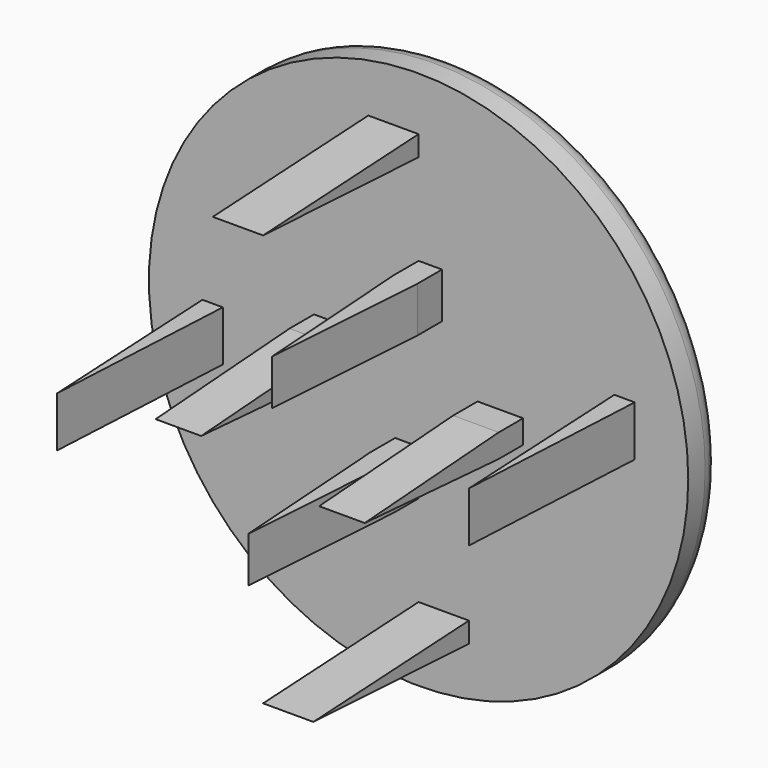
from build123d import *

# Parameters (mm, degrees)
F0_R         = 67.2715048221
F1_DEPTH     = 25.4
F2_SIZE2     = 47.9485215904
F2_SIZE      = 16.51
F3_DEPTH     = 7.62
F4_R         = 25.9737658724
F5_DEPTH     = 12.7
F6_W         = 12.5492112711
F6_H         = 5.0823129714
F6_W_2       = 5.8439155109
F6_H_2       = 11.3746980205
F6_W_3       = 5.0823129714
F6_H_3       = 12.5492112711
F6_W_4       = 11.3746980205
F6_H_4       = 5.8439155109
F7_DEPTH     = 50.8
F8_T4_DEPTH  = 276.6958225406
F8_T9_DEPTH  = 276.6958225406
F9_T4_DEPTH  = 235.8904693574
F9_T9_DEPTH  = 235.8904693574
F10_T1_DEPTH = 123.632583689
F11_T4_DEPTH = 235.8904693574
F11_T9_DEPTH = 235.8904693574
F12_T4_DEPTH = 235.8904693574
F12_T9_DEPTH = 235.8904693574
F13_T4_DEPTH = 276.6958225406
F13_T9_DEPTH = 276.6958225406
F14_T4_DEPTH = 276.6958225406
F14_T9_DEPTH = 276.6958225406
F15_T4_DEPTH = 276.6958225406
F15_T9_DEPTH = 276.6958225406
F16_R        = 5.08
F17_R        = 1.27


# Not quite as in the source:
# - a fillet or chamfer that OpenCascade refuses, or shapes differently, is made with other operations: its cross-section is extruded or revolved along the edge and cut away or added


with BuildPart() as f1:
    # F0 (on Front) → F1 (new body)
    with BuildSketch(Plane.XZ):
        Circle(F0_R)
    extrude(amount=-F1_DEPTH)

    # F2
    f2_edges = [f1.edges().sort_by_distance(p)[0] for p in [
        (-67.271505, 25.4, 0),
    ]]
    f2_side = f1.faces().sort_by_distance((-67.271505, 12.7, 0))[0]
    chamfer(f2_edges, length=F2_SIZE, length2=F2_SIZE2, reference=f2_side)

    # F3 (add): a face of the model
    f3_faces = [f1.faces().sort_by_distance(p)[0] for p in [
        (0, 25.4, 0),
    ]]
    extrude(f3_faces, amount=F3_DEPTH)

    # F4 (on face) → F5 (join)
    with BuildSketch(Plane(origin=(0, 33.02, 0), x_dir=(-1, 0, 0), z_dir=(0, 1, 0))):
        Circle(F4_R)
    extrude(amount=F5_DEPTH)

    # F6 (on face) → F7 (join)
    with BuildSketch(Plane.XZ):
        with Locations((-6.2746056356, 51.3789299875)):
            Rectangle(F6_W, F6_H)
        with Locations((2.9219577555, 20.4010321759)):
            Rectangle(F6_W_2, F6_H_2)
        with Locations((-51.3789299875, -6.2746056356)):
            Rectangle(F6_W_3, F6_H_3)
        with Locations((-20.4010321759, 2.9219577555)):
            Rectangle(F6_W_4, F6_H_4)
        with Locations((6.2746056356, -51.3789299875)):
            Rectangle(F6_W, F6_H)
        with Locations((-2.9219577555, -20.4010321759)):
            Rectangle(F6_W_2, F6_H_2)
        with Locations((51.3789299875, 6.2746056356)):
            Rectangle(F6_W_3, F6_H_3)
        with Locations((20.4010321759, -2.9219577555)):
            Rectangle(F6_W_4, F6_H_4)
    extrude(amount=F7_DEPTH)

    # F8: chamfer of 50.8 x 2.6623151876 on 2 edges, made by hand


with BuildPart() as f8_tool2:
    # F8_s3 → F8_t4 (new body)
    with BuildSketch(Plane.YZ.offset(132.0733056347)):
        Polygon((0, 53.9200864732), (-50.8, 51.2577712856), (-50.8, 53.9200864732), align=None)
    extrude(amount=-F8_T4_DEPTH)

    split(bisect_by=Plane.XZ, keep=Keep.TOP)


with BuildPart() as f1_1:
    add(f1.part)

    # F8_t1: cut F8_tool2
    add(f8_tool2.part, mode=Mode.SUBTRACT)


with BuildPart() as f8_tool7:
    # F8_s8 → F8_t9 (new body)
    with BuildSketch(Plane.YZ.offset(-144.6225169058)):
        Polygon((0, 48.8377735019), (-50.8, 51.5000886895), (-50.8, 48.8377735019), align=None)
    extrude(amount=F8_T9_DEPTH)

    split(bisect_by=Plane.XZ, keep=Keep.TOP)


with BuildPart() as f1_2:
    add(f1_1.part)

    # F8_t6: cut F8_tool7
    add(f8_tool7.part, mode=Mode.SUBTRACT)

    # F9: chamfer of 43.18 x 3.0194397397 on 2 edges, made by hand


with BuildPart() as f9_tool2:
    # F9_s3 → F9_t4 (new body)
    with BuildSketch(Plane.XY.offset(-97.5442025028)):
        Polygon((2.8244757712, -50.8), (5.8439155109, -7.62), (5.8439155109, -50.8), align=None)
    extrude(amount=F9_T4_DEPTH)

    split(bisect_by=Plane.XY.offset(-48.8377735019), keep=Keep.TOP)


with BuildPart() as f1_3:
    add(f1_2.part)

    # F9_t1: cut F9_tool2
    add(f9_tool2.part, mode=Mode.SUBTRACT)


with BuildPart() as f9_tool7:
    # F9_s8 → F9_t9 (new body)
    with BuildSketch(Plane.XY.offset(138.3462668546)):
        Polygon((3.0194397397, -50.8), (0, -7.62), (0, -50.8), align=None)
    extrude(amount=-F9_T9_DEPTH)

    split(bisect_by=Plane.XY.offset(-26.0883811861), keep=Keep.TOP)


with BuildPart() as f1_4:
    add(f1_3.part)

    # F9_t6: cut F9_tool7
    add(f9_tool7.part, mode=Mode.SUBTRACT)

    # F10: chamfer of 43.18 x 3.0194397397 on 2 edges, made by hand

    # F10_s2 → F10_t1 (cut)
    with BuildSketch(Plane.YZ.offset(-138.3462668546)):
        Polygon((-7.62, 0), (-50.8, 3.0194397397), (-50.8, 0), align=None)
        Polygon((-50.8, 2.8244757712), (-7.62, 5.8439155109), (-50.8, 5.8439155109), align=None)
    extrude(amount=F10_T1_DEPTH, mode=Mode.SUBTRACT)

    # F11: chamfer of 43.18 x 3.0194397397 on 2 edges, made by hand


with BuildPart() as f11_tool2:
    # F11_s3 → F11_t4 (new body)
    with BuildSketch(Plane.XY.offset(97.5442025028)):
        Polygon((-2.8244757712, -50.8), (-5.8439155109, -7.62), (-5.8439155109, -50.8), align=None)
    extrude(amount=-F11_T4_DEPTH)

    split(bisect_by=Plane(origin=(0, 2.5524687068, 48.7040042853), x_dir=(1, 0, 0), z_dir=(0, -0.0523359562, -0.9986295348)), keep=Keep.TOP)


with BuildPart() as f1_5:
    add(f1_4.part)

    # F11_t1: cut F11_tool2
    add(f11_tool2.part, mode=Mode.SUBTRACT)


with BuildPart() as f11_tool7:
    # F11_s8 → F11_t9 (new body)
    with BuildSketch(Plane.XY.offset(-138.3462668546)):
        Polygon((0, -7.62), (-3.0194397397, -50.8), (0, -50.8), align=None)
    extrude(amount=F11_T9_DEPTH)

    split(bisect_by=Plane(origin=(0, 2.5524687068, 48.7040042853), x_dir=(1, 0, 0), z_dir=(0, -0.0523359562, -0.9986295348)), keep=Keep.TOP)


with BuildPart() as f1_6:
    add(f1_5.part)

    # F11_t6: cut F11_tool7
    add(f11_tool7.part, mode=Mode.SUBTRACT)

    # F12: chamfer of 43.18 x 3.0194397397 on 2 edges, made by hand


with BuildPart() as f12_tool2:
    # F12_s3 → F12_t4 (new body)
    with BuildSketch(Plane.YZ.offset(-97.5442025028)):
        Polygon((-50.8, -2.8244757712), (-7.62, -5.8439155109), (-50.8, -5.8439155109), align=None)
    extrude(amount=F12_T4_DEPTH)

    split(bisect_by=Plane.YZ.offset(-48.8377735019), keep=Keep.TOP)


with BuildPart() as f1_7:
    add(f1_6.part)

    # F12_t1: cut F12_tool2
    add(f12_tool2.part, mode=Mode.SUBTRACT)


with BuildPart() as f12_tool7:
    # F12_s8 → F12_t9 (new body)
    with BuildSketch(Plane.YZ.offset(138.3462668546)):
        Polygon((-7.62, 0), (-50.8, -3.0194397397), (-50.8, 0), align=None)
    extrude(amount=-F12_T9_DEPTH)

    split(bisect_by=Plane.YZ.offset(-48.8377735019), keep=Keep.TOP)


with BuildPart() as f1_8:
    add(f1_7.part)

    # F12_t6: cut F12_tool7
    add(f12_tool7.part, mode=Mode.SUBTRACT)

    # F13: chamfer of 50.8 x 2.6623151876 on 2 edges, made by hand


with BuildPart() as f13_tool2:
    # F13_s3 → F13_t4 (new body)
    with BuildSketch(Plane.XY.offset(132.0733056347)):
        Polygon((-51.5000886895, -50.8), (-48.8377735019, 0), (-48.8377735019, -50.8), align=None)
    extrude(amount=-F13_T4_DEPTH)

    split(bisect_by=Plane.XZ, keep=Keep.TOP)


with BuildPart() as f1_9:
    add(f1_8.part)

    # F13_t1: cut F13_tool2
    add(f13_tool2.part, mode=Mode.SUBTRACT)


with BuildPart() as f13_tool7:
    # F13_s8 → F13_t9 (new body)
    with BuildSketch(Plane.XY.offset(132.0733056347)):
        Polygon((-51.2577712856, -50.8), (-53.9200864732, 0), (-53.9200864732, -50.8), align=None)
    extrude(amount=-F13_T9_DEPTH)

    split(bisect_by=Plane.XZ, keep=Keep.TOP)


with BuildPart() as f1_10:
    add(f1_9.part)

    # F13_t6: cut F13_tool7
    add(f13_tool7.part, mode=Mode.SUBTRACT)

    # F14: chamfer of 50.8 x 2.6623151876 on 2 edges, made by hand


with BuildPart() as f14_tool2:
    # F14_s3 → F14_t4 (new body)
    with BuildSketch(Plane.YZ.offset(-132.0733056347)):
        Polygon((-50.8, -51.2577712856), (0, -53.9200864732), (-50.8, -53.9200864732), align=None)
    extrude(amount=F14_T4_DEPTH)

    split(bisect_by=Plane.XZ, keep=Keep.TOP)


with BuildPart() as f1_11:
    add(f1_10.part)

    # F14_t1: cut F14_tool2
    add(f14_tool2.part, mode=Mode.SUBTRACT)


with BuildPart() as f14_tool7:
    # F14_s8 → F14_t9 (new body)
    with BuildSketch(Plane.YZ.offset(-132.0733056347)):
        Polygon((-50.8, -51.5000886895), (0, -48.8377735019), (-50.8, -48.8377735019), align=None)
    extrude(amount=F14_T9_DEPTH)

    split(bisect_by=Plane.XZ, keep=Keep.TOP)


with BuildPart() as f1_12:
    add(f1_11.part)

    # F14_t6: cut F14_tool7
    add(f14_tool7.part, mode=Mode.SUBTRACT)

    # F15: chamfer of 50.8 x 2.6623151876 on 2 edges, made by hand


with BuildPart() as f15_tool2:
    # F15_s3 → F15_t4 (new body)
    with BuildSketch(Plane.XY.offset(-132.0733056347)):
        Polygon((51.2577712856, -50.8), (53.9200864732, 0), (53.9200864732, -50.8), align=None)
    extrude(amount=F15_T4_DEPTH)

    split(bisect_by=Plane.XZ, keep=Keep.TOP)


with BuildPart() as f1_13:
    add(f1_12.part)

    # F15_t1: cut F15_tool2
    add(f15_tool2.part, mode=Mode.SUBTRACT)


with BuildPart() as f15_tool7:
    # F15_s8 → F15_t9 (new body)
    with BuildSketch(Plane.XY.offset(144.6225169058)):
        Polygon((48.8377735019, 0), (51.5000886895, -50.8), (48.8377735019, -50.8), align=None)
    extrude(amount=-F15_T9_DEPTH)

    split(bisect_by=Plane.XZ, keep=Keep.TOP)


with BuildPart() as f1_14:
    add(f1_13.part)

    # F15_t6: cut F15_tool7
    add(f15_tool7.part, mode=Mode.SUBTRACT)

    # F16
    f16_edges = [f1_14.edges().sort_by_distance(p)[0] for p in [
        (-67.271505, 8.89, 0),
    ]]
    fillet(f16_edges, radius=F16_R)

    # F17
    f17_edges = [f1_14.edges().sort_by_distance(p)[0] for p in [
        (25.973766, 45.72, 0),
        (25.973766, 33.02, 0),
    ]]
    fillet(f17_edges, radius=F17_R)


solid = f1_14.part
